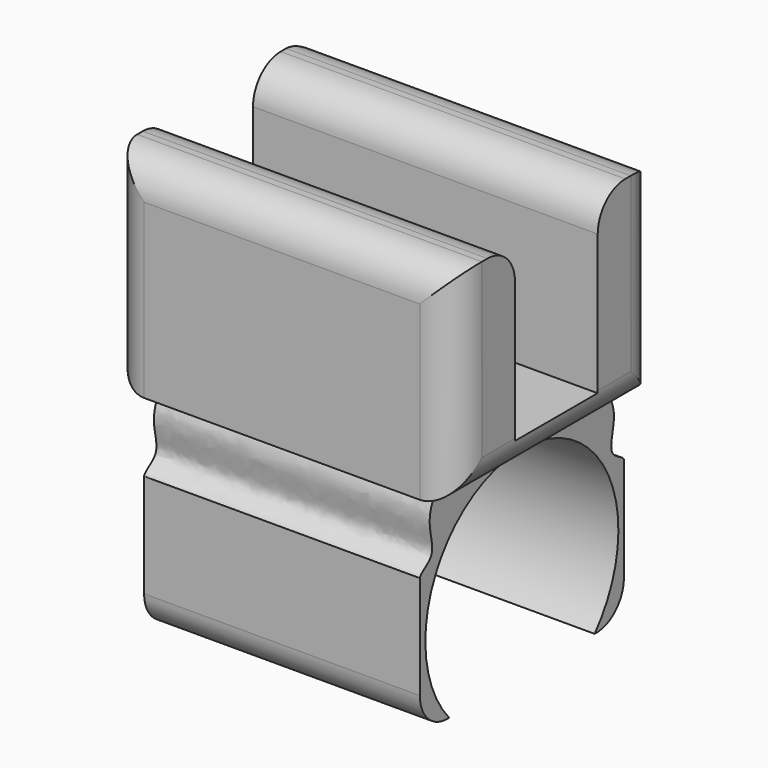
from build123d import *

# Parameters (mm, degrees)
F0_W          = 50
F0_H          = 30
F1_DEPTH      = 53
F2_W          = 15
F2_H          = 25.3311687483
F3_DEPTH      = 50.001
F4_W          = 40
F4_H          = 45
F5_DEPTH      = 10
F7_DEPTH      = 45.001
F8_DEPTH      = 20
F9_R          = 17.5
F10_DEPTH     = 45.001
F11_W         = 8
F11_H         = 30
F12_DEPTH     = 50.001
F13_TEXT_SIZE = 19.9833472107
F14_DEPTH     = 5
F15_T1_DEPTH  = 75
F15_T3_DEPTH  = 55
F15_T5_DEPTH  = 62
F15_T7_DEPTH  = 65


# Not quite as in the source:
# - a fillet or chamfer that OpenCascade refuses, or shapes differently, is made with other operations: its cross-section is extruded or revolved along the edge and cut away or added
# - Text() gives the source's letters only with a copy of the font that has no kerning and outlines rounded to 1/6400 em; it was checked with that copy


with BuildPart() as f1:
    # F0 (on Front) → F1 (new body)
    with BuildSketch(Plane.XZ):
        with Locations((0.8760225028, 0.9903833045)):
            Rectangle(F0_W, F0_H)
    extrude(amount=F1_DEPTH)

    # F2 (on face) → F3 (cut, through all)
    with BuildSketch(Plane(origin=(-24.1239774972, 0, 0), x_dir=(0, -1, 0), z_dir=(-1, 0, 0))):
        with Locations((26.5, 3.3247989304)):
            Rectangle(F2_W, F2_H)
    extrude(amount=-F3_DEPTH, mode=Mode.SUBTRACT)

    # F4 (on face) → F5 (join)
    with BuildSketch(Plane(origin=(0, 0, -14.0096166955), x_dir=(1, 0, 0), z_dir=(0, 0, -1))):
        with Locations((0.8760225028, 26.5)):
            Rectangle(F4_W, F4_H)
    extrude(amount=F5_DEPTH)

    # F6 (on face) → F7 (cut, through all)
    with BuildSketch(Plane.YZ.offset(20.8760225028)):
        with BuildLine():
            add(Edge.make_bspline(
                [(-8, -24.0096166955), (-7.9364078725, -23.4496566007), (-11.4208464018, -22.733506055), (-9.0123404283, -17.6085763796), (-10.4475317613, -15.1139475027), (-11, -14.0096166955)],
                knots=[0, 0, 0, 0, 0.2810166429, 0.6524743178, 1, 1, 1, 1], degree=3))
            Line((-8, -24.0096166955), (-4, -24.0096166955))
            Line((-4, -24.0096166955), (-4, -14.0096166955))
            Line((-4, -14.0096166955), (-11, -14.0096166955))
        make_face()
        with BuildLine():
            Line((-49, -24.0096166955), (-45, -24.0096166955))
            add(Edge.make_bspline(
                [(-45, -24.0096166955), (-44.8085905702, -23.3393763149), (-41.8872250263, -22.3681178106), (-43.7405500986, -17.9300839834), (-42.9067339422, -15.2107097876), (-42, -14.0096166955)],
                knots=[0, 0, 0, 0, 0.2915134949, 0.6402811086, 1, 1, 1, 1], degree=3))
            Line((-42, -14.0096166955), (-49, -14.0096166955))
            Line((-49, -14.0096166955), (-49, -24.0096166955))
        make_face()
    extrude(amount=-F7_DEPTH, mode=Mode.SUBTRACT)

    # F8 (add): a face of the model
    f8_faces = [f1.faces().sort_by_distance(p)[0] for p in [
        (0.8760225028, -26.5, -24.0096166955),
    ]]
    extrude(f8_faces, amount=F8_DEPTH)

    # F9 (on face) → F10 (cut, through all)
    with BuildSketch(Plane.YZ.offset(20.8760225028)):
        with Locations((-26.5, -32.5096166955)):
            Circle(F9_R)
    extrude(amount=-F10_DEPTH, mode=Mode.SUBTRACT)

    # F11 (on face) → F12 (cut, through all)
    with BuildSketch(Plane(origin=(-24.1239774972, 0, 0), x_dir=(0, -1, 0), z_dir=(-1, 0, 0))):
        with Locations((4, 0.9903833045)):
            Rectangle(F11_W, F11_H)
        with Locations((49, 0.9903833045)):
            Rectangle(F11_W, F11_H)
    extrude(amount=-F12_DEPTH, mode=Mode.SUBTRACT)

    # F13 (on face) → F14 (cut)
    with BuildSketch(Plane(origin=(0, -8, 0), x_dir=(-1, 0, 0), z_dir=(0, 1, 0))):
        with Locations((-23.3760225028, -5.8976266872)):
            Text('Mael', F13_TEXT_SIZE, font='Open Sans', text_align=(TextAlign.LEFT, TextAlign.BOTTOM))
    extrude(amount=-F14_DEPTH, mode=Mode.SUBTRACT)

    # F15: fillet of radius 5 on 12 edges, made by hand

    # F15_s2 → F15_t1 (cut)
    with BuildSketch(Plane.YZ.offset(-36.6239774972)):
        with BuildLine():
            ThreePointArc((-13, 15.9903833045), (-9.4644660941, 14.5259172104), (-8, 10.9903833045))
            Line((-8, 10.9903833045), (-8, 15.9903833045))
            Line((-8, 15.9903833045), (-13, 15.9903833045))
        make_face()
        with BuildLine():
            ThreePointArc((-45, 10.9903833045), (-43.5355339059, 14.5259172104), (-40, 15.9903833045))
            Line((-40, 15.9903833045), (-45, 15.9903833045))
            Line((-45, 15.9903833045), (-45, 10.9903833045))
        make_face()
        with BuildLine():
            ThreePointArc((-14, 15.9903833045), (-17.5355339059, 14.5259172104), (-19, 10.9903833045))
            Line((-19, 10.9903833045), (-19, 15.9903833045))
            Line((-19, 15.9903833045), (-14, 15.9903833045))
        make_face()
        with BuildLine():
            ThreePointArc((-39, 15.9903833045), (-35.4644660941, 14.5259172104), (-34, 10.9903833045))
            Line((-34, 10.9903833045), (-34, 15.9903833045))
            Line((-34, 15.9903833045), (-39, 15.9903833045))
        make_face()
    extrude(amount=F15_T1_DEPTH, mode=Mode.SUBTRACT)

    # F15_s4 → F15_t3 (cut)
    with BuildSketch(Plane.XY.offset(-26.5096166955)):
        with BuildLine():
            ThreePointArc((20.8760225028, -8), (24.4115564087, -9.4644660941), (25.8760225028, -13))
            Line((25.8760225028, -13), (25.8760225028, -8))
            Line((25.8760225028, -8), (20.8760225028, -8))
        make_face()
        with BuildLine():
            ThreePointArc((-19.1239774972, -8), (-22.6595114032, -9.4644660941), (-24.1239774972, -13))
            Line((-24.1239774972, -13), (-24.1239774972, -8))
            Line((-24.1239774972, -8), (-19.1239774972, -8))
        make_face()
        with BuildLine():
            ThreePointArc((-24.1239774972, -40), (-22.6595114032, -43.5355339059), (-19.1239774972, -45))
            Line((-19.1239774972, -45), (-24.1239774972, -45))
            Line((-24.1239774972, -45), (-24.1239774972, -40))
        make_face()
        with BuildLine():
            ThreePointArc((25.8760225028, -40), (24.4115564087, -43.5355339059), (20.8760225028, -45))
            Line((20.8760225028, -45), (25.8760225028, -45))
            Line((25.8760225028, -45), (25.8760225028, -40))
        make_face()
    extrude(amount=F15_T3_DEPTH, mode=Mode.SUBTRACT)

    # F15_s6 → F15_t5 (cut)
    with BuildSketch(Plane.XZ.offset(-4.5)):
        with BuildLine():
            ThreePointArc((25.8760225028, -9.0096166955), (24.4115564087, -12.5451506014), (20.8760225028, -14.0096166955))
            Line((20.8760225028, -14.0096166955), (25.8760225028, -14.0096166955))
            Line((25.8760225028, -14.0096166955), (25.8760225028, -9.0096166955))
        make_face()
        with BuildLine():
            ThreePointArc((-24.1239774972, -9.0096166955), (-22.6595114032, -12.5451506014), (-19.1239774972, -14.0096166955))
            Line((-19.1239774972, -14.0096166955), (-24.1239774972, -14.0096166955))
            Line((-24.1239774972, -14.0096166955), (-24.1239774972, -9.0096166955))
        make_face()
    extrude(amount=F15_T5_DEPTH, mode=Mode.SUBTRACT)

    # F15_s8 → F15_t7 (cut)
    with BuildSketch(Plane.YZ.offset(-31.6239774972)):
        with BuildLine():
            ThreePointArc((-8, -39.0096166955), (-9.4644660941, -42.5451506014), (-13, -44.0096166955))
            Line((-13, -44.0096166955), (-8, -44.0096166955))
            Line((-8, -44.0096166955), (-8, -39.0096166955))
        make_face()
        with BuildLine():
            ThreePointArc((-40, -44.0096166955), (-43.5355339059, -42.5451506014), (-45, -39.0096166955))
            Line((-45, -39.0096166955), (-45, -44.0096166955))
            Line((-45, -44.0096166955), (-40, -44.0096166955))
        make_face()
    extrude(amount=F15_T7_DEPTH, mode=Mode.SUBTRACT)


solid = f1.part
